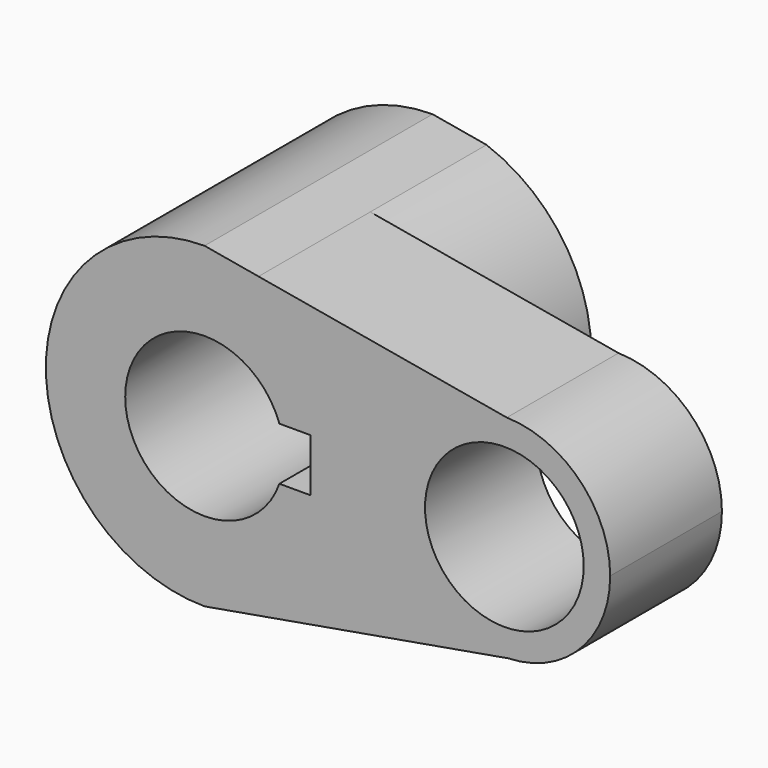
from build123d import *

# Parameters (mm, degrees)
F0_R     = 14.2875
F1_DEPTH = 25.146
F2_DEPTH = 26.162


with BuildPart() as f1:
    # F0 (on Front) → F1 (new body)
    with BuildSketch(Plane.XZ):
        with BuildLine():
            Line((9.7116618994, 26.8740441347), (0, 28.575))
            ThreePointArc((0, 28.575), (-28.575, 0), (0, -28.575))
            Line((0, -28.575), (9.6830426125, -26.8843692648))
            ThreePointArc((9.6830426125, -26.8843692648), (23.3797301915, -16.4292069551), (28.575, 0))
            ThreePointArc((28.575, 0), (23.3884732697, 16.4167579964), (9.7116618994, 26.8740441347))
        make_face()
        with BuildLine():
            ThreePointArc((-13.4703841816, 4.7625), (0, 14.2875), (13.4703841816, 4.7625))
            Line((13.4703841816, 4.7625), (19.05, 4.7625))
            Line((19.05, 4.7625), (19.05, -4.7625))
            Line((19.05, -4.7625), (13.4703841816, -4.7625))
            ThreePointArc((13.4703841816, -4.7625), (0, -14.2875), (-13.4703841816, -4.7625))
            Line((-13.4703841816, -4.7625), (-19.05, -4.7625))
            Line((-19.05, -4.7625), (-19.05, 4.7625))
            Line((-19.05, 4.7625), (-13.4703841816, 4.7625))
        make_face(mode=Mode.SUBTRACT)
        with BuildLine():
            Line((54.4119007606, 19.0449893076), (9.7116618994, 26.8740441347))
            ThreePointArc((9.7116618994, 26.8740441347), (23.3884732697, 16.4167579964), (28.575, 0))
            ThreePointArc((28.575, 0), (23.3797301915, -16.4292069551), (9.6830426125, -26.8843692648))
            Line((9.6830426125, -26.8843692648), (54.6159610506, -19.0392139788))
            ThreePointArc((54.6159610506, -19.0392139788), (34.9252734531, -0.1020710003), (54.4119007606, 19.0449893076))
        make_face()
        with BuildLine():
            ThreePointArc((73.025, 0), (67.5989762825, 13.3150204752), (54.4119007606, 19.0449893076))
            ThreePointArc((54.4119007606, 19.0449893076), (34.9252734531, -0.1020710003), (54.6159610506, -19.0392139788))
            ThreePointArc((54.6159610506, -19.0392139788), (67.6701233659, -13.241831293), (73.025, 0))
        make_face()
        with Locations((53.975, 0)):
            Circle(F0_R, mode=Mode.SUBTRACT)
        with BuildLine():
            ThreePointArc((-13.4703841816, -4.7625), (-14.2875, 0), (-13.4703841816, 4.7625))
            Line((-13.4703841816, 4.7625), (-19.05, 4.7625))
            Line((-19.05, 4.7625), (-19.05, -4.7625))
            Line((-19.05, -4.7625), (-13.4703841816, -4.7625))
        make_face()
    extrude(amount=F1_DEPTH)

    # F0 (on Front) → F2 (join)
    with BuildSketch(Plane.XZ):
        with BuildLine():
            Line((9.7116618994, 26.8740441347), (0, 28.575))
            ThreePointArc((0, 28.575), (-28.575, 0), (0, -28.575))
            Line((0, -28.575), (9.6830426125, -26.8843692648))
            ThreePointArc((9.6830426125, -26.8843692648), (23.3797301915, -16.4292069551), (28.575, 0))
            ThreePointArc((28.575, 0), (23.3884732697, 16.4167579964), (9.7116618994, 26.8740441347))
        make_face()
        with BuildLine():
            ThreePointArc((-13.4703841816, 4.7625), (0, 14.2875), (13.4703841816, 4.7625))
            Line((13.4703841816, 4.7625), (19.05, 4.7625))
            Line((19.05, 4.7625), (19.05, -4.7625))
            Line((19.05, -4.7625), (13.4703841816, -4.7625))
            ThreePointArc((13.4703841816, -4.7625), (0, -14.2875), (-13.4703841816, -4.7625))
            Line((-13.4703841816, -4.7625), (-19.05, -4.7625))
            Line((-19.05, -4.7625), (-19.05, 4.7625))
            Line((-19.05, 4.7625), (-13.4703841816, 4.7625))
        make_face(mode=Mode.SUBTRACT)
        with BuildLine():
            ThreePointArc((-13.4703841816, -4.7625), (-14.2875, 0), (-13.4703841816, 4.7625))
            Line((-13.4703841816, 4.7625), (-19.05, 4.7625))
            Line((-19.05, 4.7625), (-19.05, -4.7625))
            Line((-19.05, -4.7625), (-13.4703841816, -4.7625))
        make_face()
    extrude(amount=-F2_DEPTH)


solid = f1.part
